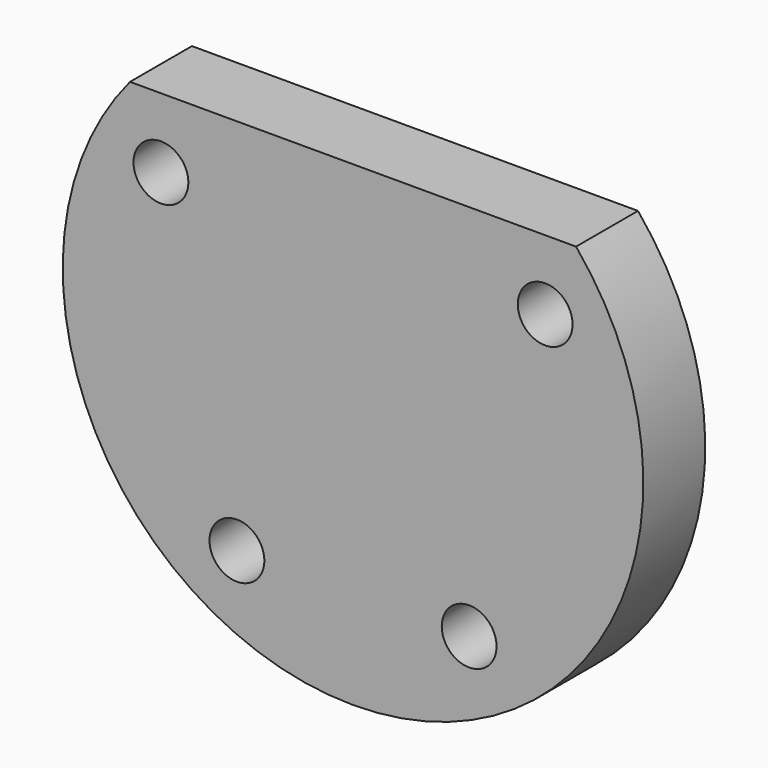
from build123d import *

# Parameters (mm, degrees)
F1_DEPTH = 6.35
F3_D     = 4.4958


with BuildPart() as f1:
    # F0 (on Front) → F1 (new body)
    with BuildSketch(Plane.XZ):
        with BuildLine():
            Line((18.2969275085, 15.24), (-18.2969275085, 15.24))
            ThreePointArc((-18.2969275085, 15.24), (0, -23.8125), (18.2969275085, 15.24))
        make_face()
    extrude(amount=F1_DEPTH)

    # F3 (through all)
    with Locations(Plane.XZ.offset(6.35)):
        with Locations((-15.7602855304, 9.525), (15.7602855304, 9.525), (9.525, -15.7602855304), (-9.525, -15.7602855304)):
            Hole(F3_D / 2)


solid = f1.part
